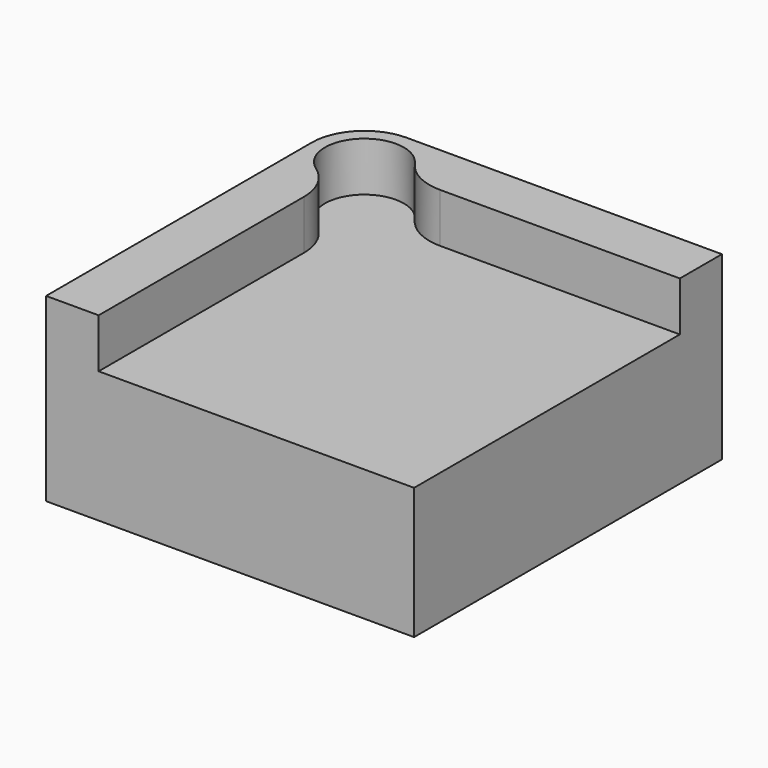
from build123d import *

# Parameters (mm, degrees)
F0_W     = 35.56
F0_H     = 37.1792408654
F1_DEPTH = 17.4625
F3_DEPTH = 4.7625
F4_R     = 5.08
F5_R     = 5.08


# Not quite as in the source:
# - a length typed as a fraction of an inch, garbled in the dataset ("3 / 203.2 mm" for 3/8 in), is restored


with BuildPart() as f1:
    # F0 (on Top) → F1 (new body)
    with BuildSketch(Plane.XY):
        Rectangle(F0_W, F0_H)
    extrude(amount=F1_DEPTH)

    # F2 (on face) → F3 (cut)
    with BuildSketch(Plane.XY.offset(17.4625)):
        with BuildLine():
            Line((-12.7, -18.5896204327), (17.78, -18.5896204327))
            Line((17.78, -18.5896204327), (17.78, 13.5096204327))
            Line((17.78, 13.5096204327), (-8.89, 13.5096204327))
            ThreePointArc((-8.89, 13.5096204327), (-15.3940768363, 16.203697269), (-12.7, 9.6996204327))
            Line((-12.7, 9.6996204327), (-12.7, -18.5896204327))
        make_face()
    extrude(amount=-F3_DEPTH, mode=Mode.SUBTRACT)

    # F4
    f4_edges = [f1.edges().sort_by_distance(p)[0] for p in [
        (-12.7, 9.69962, 15.08125),
        (-8.89, 13.50962, 15.08125),
    ]]
    fillet(f4_edges, radius=F4_R)

    # F5
    f5_edges = [f1.edges().sort_by_distance(p)[0] for p in [
        (-17.78, 18.58962, 8.73125),
    ]]
    fillet(f5_edges, radius=F5_R)


solid = f1.part
